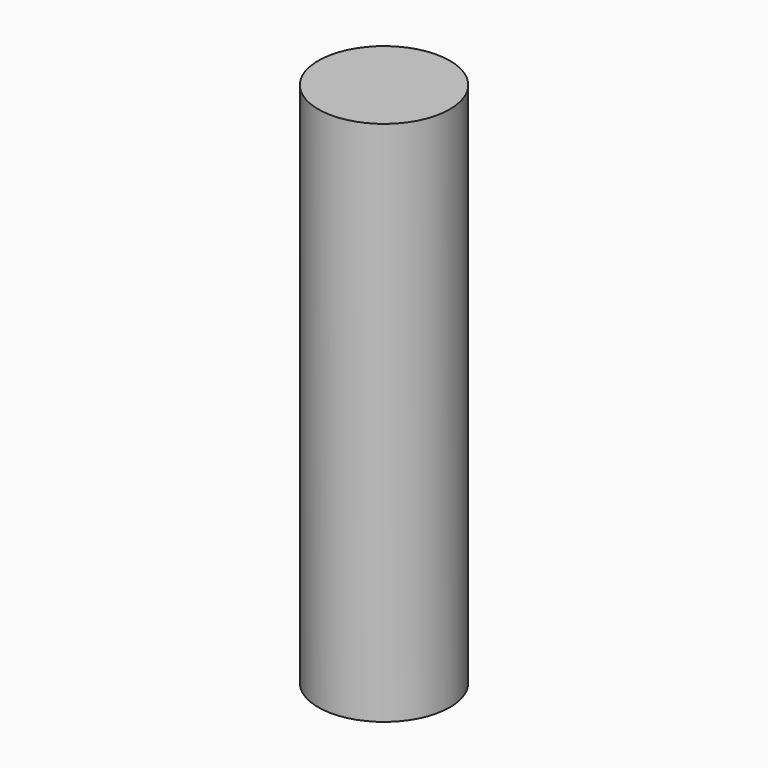
from build123d import *

# Parameters (mm, degrees)
F0_R     = 15.875
F2_DEPTH = 127


# Not quite as in the source:
# - the program builds the solid bodies; features that only make, move or delete a surface that nothing else refers to are left out


with BuildPart() as f2:
    # F0 (on Top) → F2 (new body, through all)
    with BuildSketch(Plane.XY):
        Circle(F0_R)
    extrude(amount=F2_DEPTH)


solid = f2.part
